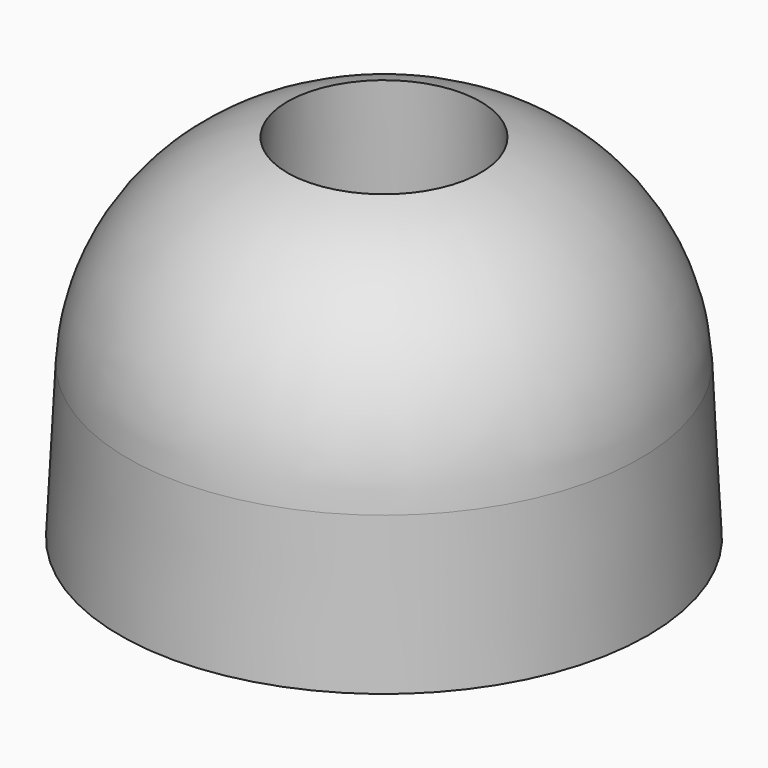
from build123d import *


# Not quite as in the source:
# - a fillet or chamfer that OpenCascade refuses, or shapes differently, is made with other operations: its cross-section is extruded or revolved along the edge and cut away or added


with BuildPart() as f1:
    # F0 (on Front) → F1 (revolve)
    with BuildSketch(Plane.XZ):
        Polygon((-22.4766174228, 36.9318798184), (-57.3878586292, 36.9318798184), (-61.4832937717, -45.2309697866), (-26.5720525653, -45.2309697866), align=None)
    revolve(axis=Axis((0, 0, 12.7753838897), (0, 0, -1)))

    # F2: fillet of radius 50.8 on 1 edges, made by hand

    # F2_s1 → F2_t2 (revolve, cut)
    with BuildSketch(Plane.XZ):
        with BuildLine():
            ThreePointArc((-22.4766174228, 36.9318798184), (-48.6034410023, 19.7340280309), (-59.7027437541, -9.5094754338))
            Line((-59.7027437541, -9.5094754338), (-57.3878586292, 36.9318798184))
            Line((-57.3878586292, 36.9318798184), (-22.4766174228, 36.9318798184))
        make_face()
    revolve(axis=Axis((0, 0, 36.9318798184), (0, 0, -1)), mode=Mode.SUBTRACT)


solid = f1.part
